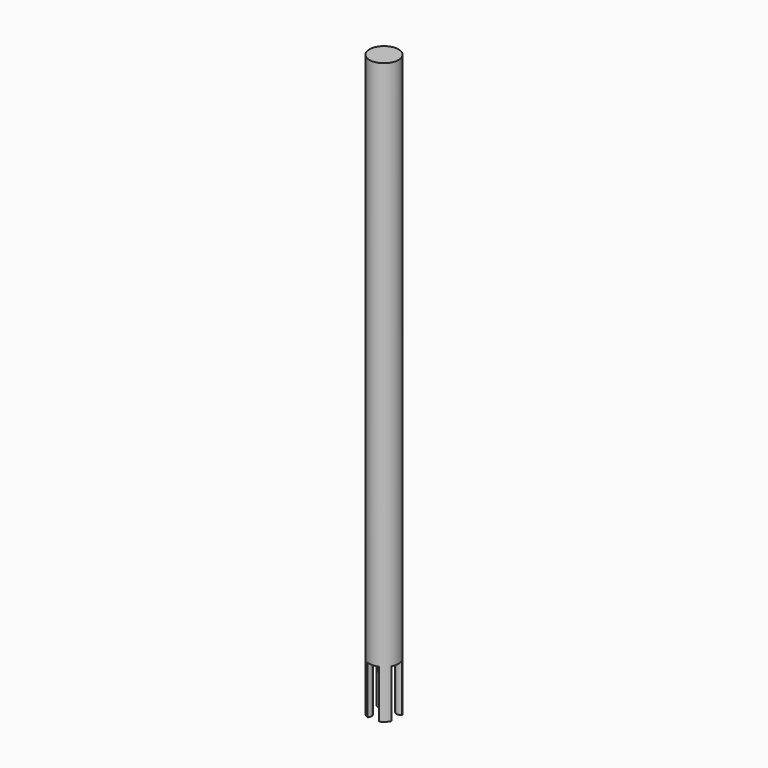
from build123d import *

# Parameters (mm, degrees)
F0_R     = 3
F1_DEPTH = 120
F3_DEPTH = 10
F4_W     = 2
F4_H     = 2
F5_DEPTH = 3
F6_R     = 0.99999


# Not quite as in the source:
# - a fillet or chamfer is up to 0.001 mm smaller than in the source, because OpenCascade refuses the exact size


with BuildPart() as f1:
    # F0 (on Top) → F1 (new body)
    with BuildSketch(Plane.XY):
        Circle(F0_R)
    extrude(amount=F1_DEPTH)

    # F2 (on face) → F3 (cut)
    with BuildSketch(Plane(origin=(0, 0, 0), x_dir=(1, 0, 0), z_dir=(0, 0, -1))):
        with BuildLine():
            ThreePointArc((-1.2, 2.749545417), (-1.2481367635, 1.3361513276), (-2.6615308529, 1.384288091))
            ThreePointArc((-2.6615308529, 1.384288091), (-3, 0), (-2.6615308529, -1.384288091))
            ThreePointArc((-2.6615308529, -1.384288091), (-1.2481367635, -1.3361513276), (-1.2, -2.749545417))
            ThreePointArc((-1.2, -2.749545417), (0, -3), (1.2, -2.749545417))
            ThreePointArc((1.2, -2.749545417), (1.2481367635, -1.3361513276), (2.6615308529, -1.384288091))
            ThreePointArc((2.6615308529, -1.384288091), (2.9141544707, -0.7125333119), (3, 0))
            ThreePointArc((3, 0), (2.9141544707, 0.7125333119), (2.6615308529, 1.384288091))
            ThreePointArc((2.6615308529, 1.384288091), (1.2481367635, 1.3361513276), (1.2, 2.749545417))
            ThreePointArc((1.2, 2.749545417), (0, 3), (-1.2, 2.749545417))
        make_face()
    extrude(amount=-F3_DEPTH, mode=Mode.SUBTRACT)

    # F4 (on face) → F5 (join)
    with BuildSketch(Plane(origin=(0, 0, 10), x_dir=(1, 0, 0), z_dir=(0, 0, -1))):
        Rectangle(F4_W, F4_H)
    extrude(amount=F5_DEPTH)

    # F6 (radius 1 in the source; OpenCascade refuses exactly that, so slightly less here)
    f6_edges = [f1.edges().sort_by_distance(p)[0] for p in [
        (0, -1, 7),
        (-1, 0, 7),
        (0, 1, 7),
        (1, 0, 7),
        (1, -1, 8.5),
        (1, 1, 8.5),
        (-1, -1, 8.5),
        (-1, 1, 8.5),
    ]]
    fillet(f6_edges, radius=F6_R)


solid = f1.part
